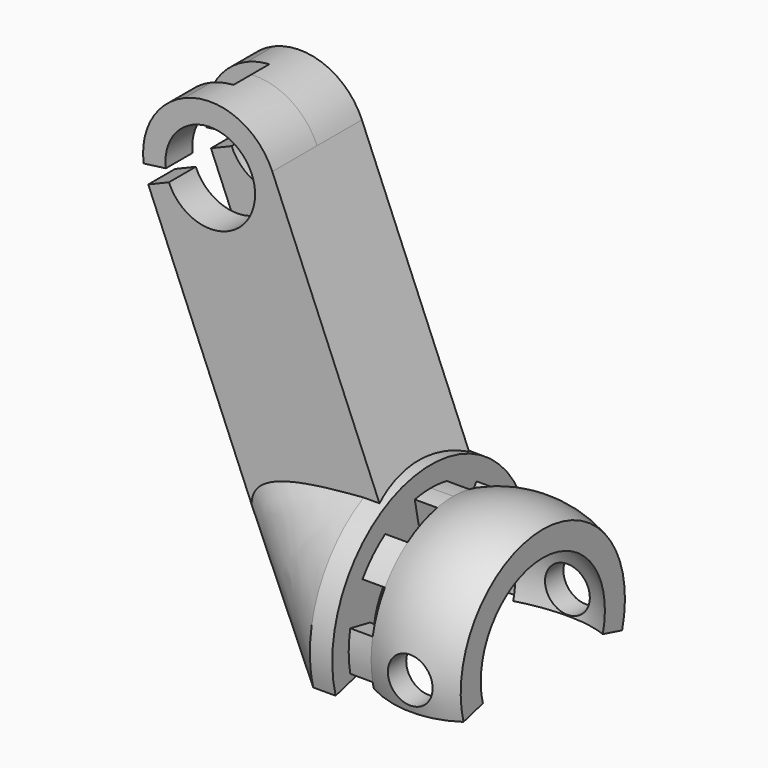
from build123d import *

# Parameters (mm, degrees)
F1_ANGLE_BACK  = 105
F1_ANGLE       = 210
F2_R           = 20
F3_DEPTH       = 100.001
F3_DEPTH_BACK  = 100.001
F5_DEPTH       = 20
F7_DEPTH       = 20
F19_DEPTH      = 110.0010001
F19_DEPTH_BACK = 110.0010001


# Not quite as in the source:
# - a feature names something its author has since deleted; it is built from what else it names


with BuildPart() as f1:
    # F0 (on Front) → F1 (revolve)
    with BuildSketch(Plane.XZ, mode=Mode.PRIVATE) as f1_sk:
        with BuildLine():
            Line((40, 69.2820323028), (40, 91.6515138991))
            ThreePointArc((40, 91.6515138991), (0, 100), (-40, 91.6515138991))
            Line((-40, 91.6515138991), (-40, 69.2820323028))
            ThreePointArc((-40, 69.2820323028), (0, 80), (40, 69.2820323028))
        make_face()
    revolve(f1_sk.sketch.rotate(Axis((77.3328692646, 0, 0), (1, 0, 0)), -F1_ANGLE_BACK), axis=Axis((77.3328692646, 0, 0), (1, 0, 0)), revolution_arc=F1_ANGLE)

    # F2 (on Front) → F3 (cut, two sides)
    with BuildSketch(Plane.XZ) as f3_sk:
        Circle(F2_R)
    extrude(amount=-F3_DEPTH, mode=Mode.SUBTRACT)
    extrude(f3_sk.sketch, amount=F3_DEPTH_BACK, mode=Mode.SUBTRACT)

    # F4 (on face) → F5 (join)
    with BuildSketch(Plane(origin=(-40, 0, 0), x_dir=(0, -1, 0), z_dir=(-1, 0, 0))):
        with BuildLine():
            Line((0, 91.6515138991), (0, 69.2820323028))
            ThreePointArc((0, 69.2820323028), (6.7908266825, 68.9484203805), (13.5162539919, 67.950797479))
            Line((13.5162539919, 67.950797479), (17.8803233598, 89.8904557589))
            ThreePointArc((17.8803233598, 89.8904557589), (8.9834192993, 91.2101868088), (0, 91.6515138991))
        make_face()
        with BuildLine():
            ThreePointArc((-57.6059045383, 38.4910348305), (-48.9897948557, 48.9897948557), (-38.4910348305, 57.6059045383))
            Line((-38.4910348305, 57.6059045383), (-50.9188529335, 76.2054487286))
            ThreePointArc((-50.9188529335, 76.2054487286), (-64.8074069841, 64.8074069841), (-76.2054487286, 50.9188529335))
            Line((-76.2054487286, 50.9188529335), (-57.6059045383, 38.4910348305))
        make_face()
        with BuildLine():
            ThreePointArc((-67.950797479, -13.5162539919), (-69.2820323028, 0), (-67.950797479, 13.5162539919))
            Line((-67.950797479, 13.5162539919), (-89.8904557589, 17.8803233598))
            ThreePointArc((-89.8904557589, 17.8803233598), (-91.6515138991, 0), (-89.8904557589, -17.8803233598))
            Line((-89.8904557589, -17.8803233598), (-67.950797479, -13.5162539919))
        make_face()
        with BuildLine():
            Line((50.9188529335, 76.2054487286), (38.4910348305, 57.6059045383))
            ThreePointArc((38.4910348305, 57.6059045383), (48.9897948557, 48.9897948557), (57.6059045383, 38.4910348305))
            Line((57.6059045383, 38.4910348305), (76.2054487286, 50.9188529335))
            ThreePointArc((76.2054487286, 50.9188529335), (64.8074069841, 64.8074069841), (50.9188529335, 76.2054487286))
        make_face()
        with BuildLine():
            ThreePointArc((-13.5162539919, 67.950797479), (-6.7908266825, 68.9484203805), (0, 69.2820323028))
            Line((0, 69.2820323028), (0, 91.6515138991))
            ThreePointArc((0, 91.6515138991), (-8.9834192993, 91.2101868088), (-17.8803233598, 89.8904557589))
            Line((-17.8803233598, 89.8904557589), (-13.5162539919, 67.950797479))
        make_face()
        with BuildLine():
            Line((89.8904557589, 17.8803233598), (67.950797479, 13.5162539919))
            ThreePointArc((67.950797479, 13.5162539919), (68.9484203805, 6.7908266825), (69.2820323028, 0))
            ThreePointArc((69.2820323028, 0), (68.9484203805, -6.7908266825), (67.950797479, -13.5162539919))
            Line((67.950797479, -13.5162539919), (89.8904557589, -17.8803233598))
            ThreePointArc((89.8904557589, -17.8803233598), (91.6515138991, 0), (89.8904557589, 17.8803233598))
        make_face()
    extrude(amount=F5_DEPTH)

    # F6 (on face) → F7 (join)
    with BuildSketch(Plane(origin=(-60, 0, 0), x_dir=(0, -1, 0), z_dir=(-1, 0, 0))):
        with BuildLine():
            Line((61.8192528825, -16.5644188866), (106.2518408918, -28.4700949613))
            ThreePointArc((106.2518408918, -28.4700949613), (0, 110), (-106.2518408918, -28.4700949613))
            Line((-106.2518408918, -28.4700949613), (-61.8192528825, -16.5644188866))
            ThreePointArc((-61.8192528825, -16.5644188866), (0, 64), (61.8192528825, -16.5644188866))
        make_face()
    extrude(amount=F7_DEPTH)

    # F7_face (on face) → F11 section 0
    with BuildSketch(Plane(origin=(-80, 0, 46.9243182834), x_dir=(0, -1, 0), z_dir=(-1, 0, 0))):
        with BuildLine():
            Line((-106.2518408918, -75.3944132447), (-61.8192528825, -63.4887371699))
            ThreePointArc((-61.8192528825, -63.4887371699), (0, 17.0756817166), (61.8192528825, -63.4887371699))
            Line((61.8192528825, -63.4887371699), (106.2518408918, -75.3944132447))
            ThreePointArc((106.2518408918, -75.3944132447), (0, 63.0756817166), (-106.2518408918, -75.3944132447))
        make_face()
    # F9 (on offset) → F11 section 1
    with BuildSketch(Plane(origin=(-180, 0, 0), x_dir=(0, -1, 0), z_dir=(-1, 0, 0))):
        with BuildLine():
            Line((20, 60), (50, 60))
            ThreePointArc((50, 60), (0, 110), (-50, 60))
            Line((-50, 60), (-20, 60))
            ThreePointArc((-20, 60), (0, 80), (20, 60))
        make_face()
    loft()

    # F16 (on face) → F17 (join, up to the next surface of F1)
    with BuildSketch(Plane(origin=(-163.3136094675, 0, 391.9526627219), x_dir=(0.9230769231, 0, 0.3846153846), z_dir=(-0.3846153846, 0, 0.9230769231))):
        Polygon((-143.0769230769, -20), (-143.0769230769, -50), (-23.0769230769, -50), (-23.0769230769, 50), (-143.0769230769, 50), (-143.0769230769, 20), (-63.0769230769, 20), (-63.0769230769, -20), align=None)
    extrude(until=Until.NEXT, dir=(0.3846153846, 0, -0.9230769231))

    # F18 (on Front) → F19 (cut, two sides)
    with BuildSketch(Plane.XZ) as f19_sk:
        with BuildLine():
            Line((-295.3846153846, 336.9230769231), (-272.3076923077, 281.5384615385))
            ThreePointArc((-272.3076923077, 281.5384615385), (-274.8460121427, 288.9650307682), (-276.3932544968, 296.6593818913))
            ThreePointArc((-276.3932544968, 296.6593818913), (-268.9472491257, 334.5066125365), (-240.0000021838, 359.9999990901))
            Line((-240.0000021838, 359.9999990901), (-295.3846153846, 336.9230769231))
        make_face()
        with BuildLine():
            ThreePointArc((-240.0000021838, 359.9999990901), (-194.0780897016, 360.0960709742), (-161.5384615385, 327.6923076923))
            Line((-161.5384615385, 327.6923076923), (-184.6153846154, 383.0769230769))
            Line((-184.6153846154, 383.0769230769), (-240.0000021838, 359.9999990901))
        make_face()
        with BuildLine():
            Line((-216.9230769231, 304.6153846154), (-180, 320))
            ThreePointArc((-180, 320), (-227.3566461545, 343.2306747618), (-256.5698619723, 299.3113827993))
            Line((-256.5698619723, 299.3113827993), (-216.9230769231, 304.6153846154))
        make_face()
        with BuildLine():
            ThreePointArc((-256.5698619723, 299.3113827993), (-255.5383670695, 294.1818153839), (-253.8461538462, 289.2307692308))
            Line((-253.8461538462, 289.2307692308), (-216.9230769231, 304.6153846154))
            Line((-216.9230769231, 304.6153846154), (-256.5698619723, 299.3113827993))
        make_face()
        with BuildLine():
            ThreePointArc((-253.8461538462, 289.2307692308), (-209.0784315175, 265.3921575877), (-176.9230769231, 304.6153846154))
            ThreePointArc((-176.9230769231, 304.6153846154), (-177.6998498954, 312.4600300209), (-180, 320))
            Line((-180, 320), (-216.9230769231, 304.6153846154))
            Line((-216.9230769231, 304.6153846154), (-253.8461538462, 289.2307692308))
        make_face()
        with BuildLine():
            Line((-272.3076923077, 281.5384615385), (-253.8461538462, 289.2307692308))
            ThreePointArc((-253.8461538462, 289.2307692308), (-255.5383670695, 294.1818153839), (-256.5698619723, 299.3113827993))
            Line((-256.5698619723, 299.3113827993), (-276.3932544968, 296.6593818913))
            ThreePointArc((-276.3932544968, 296.6593818913), (-274.8460121427, 288.9650307682), (-272.3076923077, 281.5384615385))
        make_face()
    extrude(amount=-F19_DEPTH, mode=Mode.SUBTRACT)
    extrude(f19_sk.sketch, amount=F19_DEPTH_BACK, mode=Mode.SUBTRACT)


solid = f1.part
